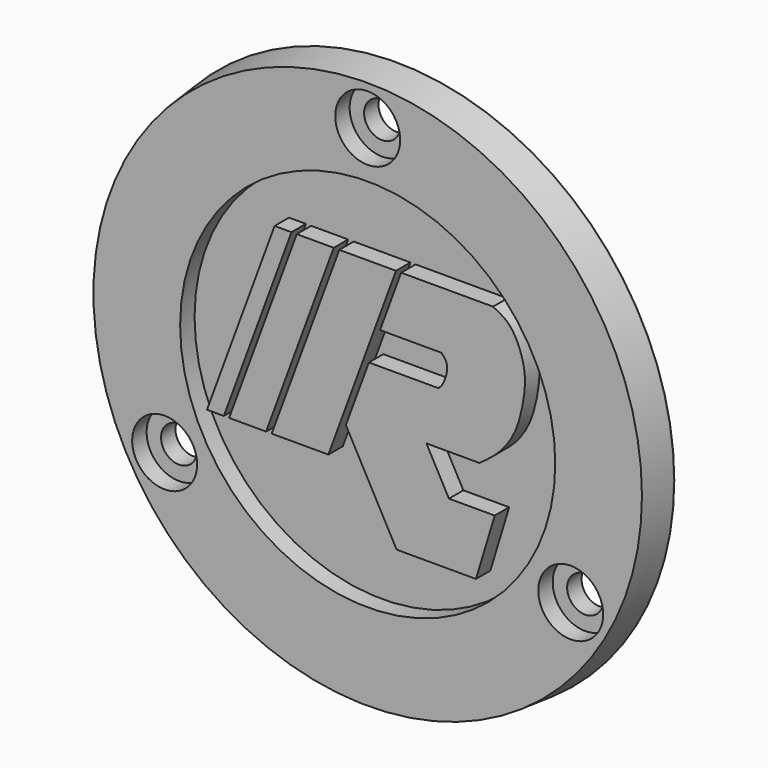
from build123d import *

# Parameters (mm, degrees)
F0_R            = 48.895
F1_DEPTH        = 6.35
F2_R            = 33.02
F3_DEPTH        = 3.175
F4_R            = 3.175
F5_DEPTH        = 6.351
F5_COPIES_COUNT = 3
F6_R            = 5.715
F7_DEPTH        = 3.175
F9_DEPTH        = 3.175


# Not quite as in the source:
# - a pattern or mirror of a feature is missing from the dataset's text; its kind, count and spacing are read off the source's solid


with BuildPart() as f1:
    # F0 (on Front) → F1 (new body)
    with BuildSketch(Plane.XZ):
        Circle(F0_R)
    extrude(amount=F1_DEPTH)

    # F2 (on face) → F3 (cut)
    with BuildSketch(Plane.XZ.offset(6.35)):
        Circle(F2_R)
    extrude(amount=-F3_DEPTH, mode=Mode.SUBTRACT)

    # F4 (on face) → F5 (cut, through all)
    with BuildSketch(Plane.XZ.offset(6.35)):
        with Locations((0, 41.275)):
            Circle(F4_R)
    f5 = extrude(amount=-F5_DEPTH, mode=Mode.SUBTRACT)

    # F5_copies: F5 ×3 about axis
    f5_copies_axis = Axis((0, 0, 0), (0, 1, 0))
    for i in range(1, F5_COPIES_COUNT):
        add(f5.rotate(f5_copies_axis, i * 360 / F5_COPIES_COUNT), mode=Mode.SUBTRACT)

    # F6 (on face) → F7 (cut)
    with BuildSketch(Plane.XZ.offset(6.35)):
        with Locations((0, 41.275)):
            Circle(F6_R)
        with Locations((35.7451985412, -20.6375)):
            Circle(F6_R)
        with Locations((-35.7451985412, -20.6375)):
            Circle(F6_R)
    extrude(amount=-F7_DEPTH, mode=Mode.SUBTRACT)

    # F8 (on face) → F9 (join)
    with BuildSketch(Plane.XZ.offset(3.175)):
        Polygon((-16.3922007191, 20.7727154884), (-28.2979620914, -11.5829327573), (-25.324323939, -11.5829327573), (-13.4185625667, 20.7727154884), align=None)
        Polygon((-16.905579319, -11.5829327573), (-6.9219360217, -11.5829327573), (4.9838253506, 20.7727154884), (-4.9998179467, 20.7727154884), align=None)
        Polygon((-12.4935675046, 20.7727154884), (-24.3993288769, -11.5829327573), (-17.8866158386, -11.5829327573), (-5.9808544663, 20.7727154884), align=None)
        with BuildLine():
            Line((5.8897674028, 20.7727154884), (2.173845637, 10.6741544806))
            Line((2.173845637, 10.6741544806), (12.9963092812, 10.6741544806))
            add(Edge.make_bspline(
                [(12.9963092812, 10.6741544806), (13.3555097893, 10.2684161805), (14.1043976934, 9.4225028304), (13.9491779559, 7.5181571268), (13.1134705599, 5.5267271878), (12.6059829763, 5.1538653523), (12.4124220311, 5.0116520418)],
                knots=[0, 0, 0, 0, 0.2524611124, 0.5263496824, 0.8193449335, 1, 1, 1, 1], degree=3))
            Line((12.4124220311, 5.0116520418), (0.2083620148, 5.0116520418))
            Line((0.2083620148, 5.0116520418), (-3.8432038956, -5.9990710312))
            Line((-3.8432038956, -5.9990710312), (5.090538634, -22.4072845116))
            Line((5.090538634, -22.4072845116), (19.059962988, -22.4072845116))
            Line((19.059962988, -22.4072845116), (22.3604289031, -11.5080620742))
            Line((22.3604289031, -11.5080620742), (14.3011480982, -11.5080620742))
            Line((14.3011480982, -11.5080620742), (10.3404486879, -4.2336190018))
            Line((10.3404486879, -4.2336190018), (19.6740036189, -4.2336190018))
            add(Edge.make_bspline(
                [(22.0640265758, 20.7727154884), (22.9280250832, 20.3392576633), (24.6989276358, 19.4508168126), (26.5202053139, 16.7535424772), (27.942801324, 12.3470202028), (27.4780031336, 7.7394644811), (26.2592507252, 2.6453616364), (23.4242960391, -1.5113689868), (20.9094052375, -3.3368697093), (19.6740036189, -4.2336190018)],
                knots=[0, 0, 0, 0, 0.1175129286, 0.2408614638, 0.3885970952, 0.5383784175, 0.6968239202, 0.8510693906, 1, 1, 1, 1], degree=3))
            Line((22.0640265758, 20.7727154884), (5.8897674028, 20.7727154884))
        make_face()
    extrude(amount=F9_DEPTH)

    # F10 (on Top) → F11 (revolve, cut)
    with BuildSketch(Plane.XY):
        Polygon((48.9125326276, -6.3948447905), (48.9125326276, 0), (48.2775326276, -6.3948447905), align=None)
    revolve(axis=Axis((0, -3.4167582635, 0), (0, -1, 0)), mode=Mode.SUBTRACT)


solid = f1.part
